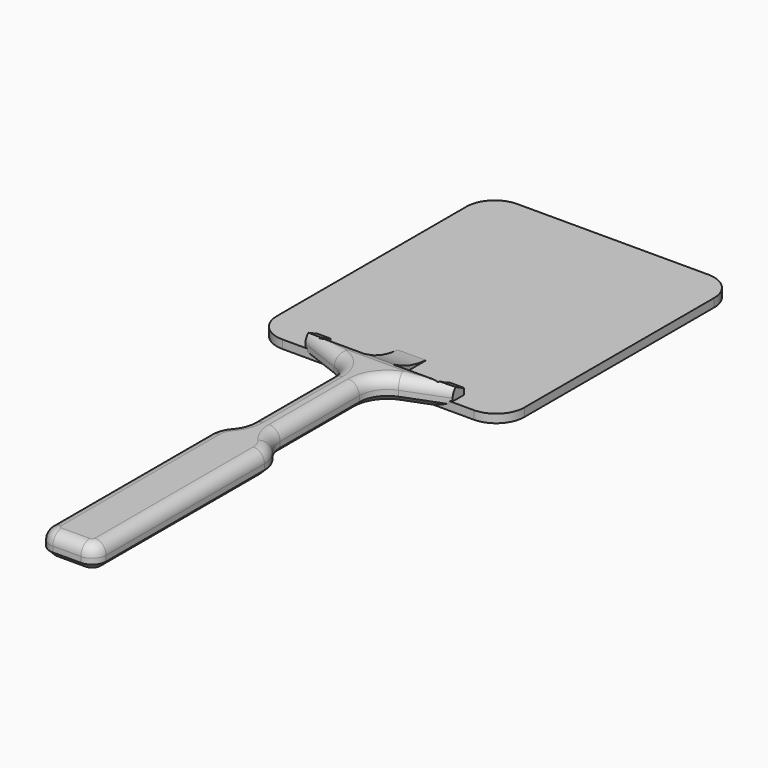
from build123d import *

# Parameters (mm, degrees)
F2_DEPTH      = 3
F1_W          = 10
F1_H          = 50.7820645242
F1_H_2        = 8.1103595249
F1_H_3        = 14.6
F1_W_2        = 5
F1_H_4        = 5
F3_DEPTH      = 8
F4_T1_DEPTH   = 8
F5_R          = 10
F6_R          = 5
F7_R          = 10
F8_R          = 31.9895246327
F9_DEPTH      = 30
F9_DEPTH_BACK = 30
F10_T1_DEPTH  = 44.710583772
F10_T3_DEPTH  = 55.9785297761
F10_T5_DEPTH  = 44.710583772
F10_T7_DEPTH  = 35.23873089
F10_T9_DEPTH  = 70.4314974826
F10_T11_DEPTH = 10
F10_T14_ANGLE = 69.0798918948
F10_T16_ANGLE = 69.0798918948
F10_T18_ANGLE = 41.4096221077
F10_T20_ANGLE = 41.4096221088
F10_T22_ANGLE = 90
F10_T24_ANGLE = 90
F10_T26_ANGLE = 41.4096221088
F10_T28_ANGLE = 41.4096221077
F11_T1_DEPTH  = 70.4314974826
F11_T3_DEPTH  = 35.23873089
F11_T5_DEPTH  = 20.9741913293
F11_T7_DEPTH  = 10
F11_T9_DEPTH  = 20.9741913293
F11_T12_ANGLE = 69.0798918948
F11_T14_ANGLE = 41.4096221077
F11_T16_ANGLE = 41.4096221088
F11_T18_ANGLE = 90
F11_T20_ANGLE = 90
F11_T22_ANGLE = 41.4096221088
F11_T24_ANGLE = 41.4096221077
F11_T26_ANGLE = 69.0798918948


# Not quite as in the source:
# - a fillet or chamfer that OpenCascade refuses, or shapes differently, is made with other operations: its cross-section is extruded or revolved along the edge and cut away or added


with BuildPart() as f2:
    # F0 (on Top) → F2 (new body)
    with BuildSketch(Plane.XY):
        with BuildLine():
            Line((34.0520262078, 104.4403978414), (-34.0520262078, 104.4403978414))
            ThreePointArc((-34.0520262078, 104.4403978414), (-41.1230940197, 101.5114656532), (-44.0520262078, 94.4403978414))
            Line((-44.0520262078, 94.4403978414), (-44.0520262078, 10))
            ThreePointArc((-44.0520262078, 10), (-41.1230940197, 2.9289321881), (-34.0520262078, 0))
            Line((-34.0520262078, 0), (34.0520262078, 0))
            ThreePointArc((34.0520262078, 0), (41.1230940197, 2.9289321881), (44.0520262078, 10))
            Line((44.0520262078, 10), (44.0520262078, 94.4403978414))
            ThreePointArc((44.0520262078, 94.4403978414), (41.1230940197, 101.5114656532), (34.0520262078, 104.4403978414))
        make_face()
    extrude(amount=F2_DEPTH)


with BuildPart() as f3:
    # F1 (on Top) → F3 (new body)
    with BuildSketch(Plane.XY):
        Polygon((5, -58.4924240492), (-5, -58.4924240492), (-10, -58.4924240492), (-10, -138.4924240492), (10, -138.4924240492), (10, -58.4924240492), align=None)
        with Locations((0, -33.1013917871)):
            Rectangle(F1_W, F1_H)
        with Locations((0, -3.6551797625)):
            Rectangle(F1_W, F1_H_2)
        Polygon((-5, -7.7103595249), (-5, 0.4), (-21.2165865879, 0.4), (-26.2165865879, 0.4), align=None)
        Polygon((21.2165865879, 0.4), (5, 0.4), (5, -7.7103595249), (26.2165865879, 0.4), align=None)
        with Locations((0, 7.7)):
            Rectangle(F1_W, F1_H_3)
        with Locations((-23.7165865879, 2.9)):
            Rectangle(F1_W_2, F1_H_4)
        with Locations((23.7165865879, 2.9)):
            Rectangle(F1_W_2, F1_H_4)
    extrude(amount=F3_DEPTH)

    # F4: fillet of radius 10 on 2 edges, made by hand

    # F4_s2 → F4_t1 (join)
    with BuildSketch(Plane.XY):
        with BuildLine():
            ThreePointArc((-10, -58.4924240492), (-6.3397459622, -54.8321700113), (-5, -49.8321700113))
            Line((-5, -49.8321700113), (-5, -58.4924240492))
            Line((-5, -58.4924240492), (-10, -58.4924240492))
        make_face()
        with BuildLine():
            ThreePointArc((10, -58.4924240492), (6.3397459622, -54.8321700113), (5, -49.8321700113))
            Line((5, -49.8321700113), (5, -58.4924240492))
            Line((5, -58.4924240492), (10, -58.4924240492))
        make_face()
    extrude(amount=F4_T1_DEPTH)

    # F5
    f5_edges = [f3.edges().sort_by_distance(p)[0] for p in [
        (10, -58.492424, 4),
        (-10, -58.492424, 4),
    ]]
    fillet(f5_edges, radius=F5_R)

    # F6
    f6_edges = [f3.edges().sort_by_distance(p)[0] for p in [
        (-10, -138.492424, 4),
        (10, -138.492424, 4),
    ]]
    fillet(f6_edges, radius=F6_R)

    # F7
    f7_edges = [f3.edges().sort_by_distance(p)[0] for p in [
        (-5, -7.71036, 4),
        (5, -7.71036, 4),
    ]]
    fillet(f7_edges, radius=F7_R)

    # F8 (on Right) → F9 (cut, two sides)
    with BuildSketch(Plane.YZ) as f9_sk:
        with Locations((17.1725142692, 34.9895246327)):
            Circle(F8_R)
    extrude(amount=-F9_DEPTH, mode=Mode.SUBTRACT)
    extrude(f9_sk.sketch, amount=F9_DEPTH_BACK, mode=Mode.SUBTRACT)

    # F10: fillet of radius 4 on 16 edges, made by hand

    # F10_s2 → F10_t1 (cut)
    with BuildSketch(Plane(origin=(-49.9834696062, 19.1069334895, 0), x_dir=(0, 0, 1), z_dir=(0.9340792186, -0.3570658389, 0))):
        with BuildLine():
            ThreePointArc((4, 8.9874157949), (6.8284271247, 7.8158429197), (8, 4.9874157949))
            Line((8, 4.9874157949), (8, 8.9874157949))
            Line((8, 8.9874157949), (4, 8.9874157949))
        make_face()
    extrude(amount=F10_T1_DEPTH, mode=Mode.SUBTRACT)

    # F10_s4 → F10_t3 (cut)
    with BuildSketch(Plane.YZ.offset(-27.9892648881)):
        with BuildLine():
            ThreePointArc((-1.1276290725, 8), (-0.0733831244, 7.8585703934), (0.9063120288, 7.4442827405))
            ThreePointArc((0.9063120288, 7.4442827405), (0.4508473107, 7.7183761355), (0, 8))
            Line((0, 8), (-1.1276290725, 8))
        make_face()
    extrude(amount=F10_T3_DEPTH, mode=Mode.SUBTRACT)

    # F10_s6 → F10_t5 (cut)
    with BuildSketch(Plane(origin=(8.2202424512, 3.1423113885, 0), x_dir=(0, 0, 1), z_dir=(0.9340792186, 0.3570658389, 0))):
        with BuildLine():
            ThreePointArc((4, 8.9874157949), (6.8284271247, 7.8158429197), (8, 4.9874157949))
            Line((8, 4.9874157949), (8, 8.9874157949))
            Line((8, 8.9874157949), (4, 8.9874157949))
        make_face()
    extrude(amount=F10_T5_DEPTH, mode=Mode.SUBTRACT)

    # F10_s8 → F10_t7 (cut)
    with BuildSketch(Plane.XZ.offset(14.5934391213)):
        with BuildLine():
            ThreePointArc((5, 4), (3.8284271247, 6.8284271247), (1, 8))
            Line((1, 8), (5, 8))
            Line((5, 8), (5, 4))
        make_face()
        with BuildLine():
            ThreePointArc((-5, 4), (-3.8284271247, 6.8284271247), (-1, 8))
            Line((-1, 8), (-5, 8))
            Line((-5, 8), (-5, 4))
        make_face()
    extrude(amount=F10_T7_DEPTH, mode=Mode.SUBTRACT)

    # F10_s10 → F10_t9 (cut)
    with BuildSketch(Plane.XZ.offset(63.0609265666)):
        with BuildLine():
            ThreePointArc((10, 4), (8.8284271247, 6.8284271247), (6, 8))
            Line((6, 8), (10, 8))
            Line((10, 8), (10, 4))
        make_face()
        with BuildLine():
            ThreePointArc((-10, 4), (-8.8284271247, 6.8284271247), (-6, 8))
            Line((-6, 8), (-10, 8))
            Line((-10, 8), (-10, 4))
        make_face()
    extrude(amount=F10_T9_DEPTH, mode=Mode.SUBTRACT)

    # F10_s12 → F10_t11 (cut)
    with BuildSketch(Plane.YZ.offset(-5)):
        with BuildLine():
            ThreePointArc((-138.4924240492, 4), (-137.3208511739, 6.8284271247), (-134.4924240492, 8))
            Line((-134.4924240492, 8), (-138.4924240492, 8))
            Line((-138.4924240492, 8), (-138.4924240492, 4))
        make_face()
    extrude(amount=F10_T11_DEPTH, mode=Mode.SUBTRACT)

    # F10_s13 → F10_t14 (revolve, cut)
    with BuildSketch(Plane.XZ.offset(14.5934391213)):
        with BuildLine():
            ThreePointArc((-5, 4), (-3.8284271247, 6.8284271247), (-1, 8))
            Line((-1, 8), (-5, 8))
            Line((-5, 8), (-5, 4))
        make_face()
    revolve(axis=Axis((-15, -14.5934391213, 8), (0, 0, 1)), revolution_arc=F10_T14_ANGLE, mode=Mode.SUBTRACT)

    # F10_s15 → F10_t16 (revolve, cut)
    with BuildSketch(Plane.XZ.offset(14.5934391213)):
        with BuildLine():
            ThreePointArc((5, 4), (3.8284271247, 6.8284271247), (1, 8))
            Line((1, 8), (5, 8))
            Line((5, 8), (5, 4))
        make_face()
    revolve(axis=Axis((15, -14.5934391213, 8), (0, 0, -1)), revolution_arc=F10_T16_ANGLE, mode=Mode.SUBTRACT)

    # F10_s17 → F10_t18 (revolve, cut)
    with BuildSketch(Plane(origin=(31.2831617138, -35.4717711942, 0), x_dir=(0, 0, 1), z_dir=(0.6614378278, -0.75, 0))):
        with BuildLine():
            ThreePointArc((4, 31.7108822847), (6.8284271247, 32.88245516), (8, 35.7108822847))
            Line((8, 35.7108822847), (8, 31.7108822847))
            Line((8, 31.7108822847), (4, 31.7108822847))
        make_face()
    revolve(axis=Axis((15.0000000004, -49.8321700111, 8), (0, 0, -1)), revolution_arc=F10_T18_ANGLE, mode=Mode.SUBTRACT)

    # F10_s19 → F10_t20 (revolve, cut)
    with BuildSketch(Plane.XZ.offset(63.0609265666)):
        with BuildLine():
            ThreePointArc((10, 4), (8.8284271247, 6.8284271247), (6, 8))
            Line((6, 8), (10, 8))
            Line((10, 8), (10, 4))
        make_face()
    revolve(axis=Axis((0, -63.0609265666, 8), (0, 0, 1)), revolution_arc=F10_T20_ANGLE, mode=Mode.SUBTRACT)

    # F10_s21 → F10_t22 (revolve, cut)
    with BuildSketch(Plane.YZ.offset(5)):
        with BuildLine():
            ThreePointArc((-138.4924240492, 4), (-137.3208511739, 6.8284271247), (-134.4924240492, 8))
            Line((-134.4924240492, 8), (-138.4924240492, 8))
            Line((-138.4924240492, 8), (-138.4924240492, 4))
        make_face()
    revolve(axis=Axis((5, -133.4924240492, 8), (0, 0, 1)), revolution_arc=F10_T22_ANGLE, mode=Mode.SUBTRACT)

    # F10_s23 → F10_t24 (revolve, cut)
    with BuildSketch(Plane.XZ.offset(133.4924240492)):
        with BuildLine():
            ThreePointArc((-10, 4), (-8.8284271247, 6.8284271247), (-6, 8))
            Line((-6, 8), (-10, 8))
            Line((-10, 8), (-10, 4))
        make_face()
    revolve(axis=Axis((-5, -133.4924240492, 8), (0, 0, 1)), revolution_arc=F10_T24_ANGLE, mode=Mode.SUBTRACT)

    # F10_s25 → F10_t26 (revolve, cut)
    with BuildSketch(Plane.XZ.offset(63.0609265666)):
        with BuildLine():
            ThreePointArc((-10, 4), (-8.8284271247, 6.8284271247), (-6, 8))
            Line((-6, 8), (-10, 8))
            Line((-10, 8), (-10, 4))
        make_face()
    revolve(axis=Axis((0, -63.0609265666, 8), (0, 0, -1)), revolution_arc=F10_T26_ANGLE, mode=Mode.SUBTRACT)

    # F10_s27 → F10_t28 (revolve, cut)
    with BuildSketch(Plane(origin=(-31.2831617138, -35.4717711942, 0), x_dir=(0, 0, 1), z_dir=(-0.6614378278, -0.75, 0))):
        with BuildLine():
            ThreePointArc((4, -31.7108822847), (6.8284271247, -32.88245516), (8, -35.7108822847))
            Line((8, -35.7108822847), (8, -31.7108822847))
            Line((8, -31.7108822847), (4, -31.7108822847))
        make_face()
    revolve(axis=Axis((-15.0000000004, -49.8321700111, 8), (0, 0, 1)), revolution_arc=F10_T28_ANGLE, mode=Mode.SUBTRACT)

    # F11: chamfer of 2 on 15 edges, made by hand

    # F11_s2 → F11_t1 (cut)
    with BuildSketch(Plane.XZ.offset(63.0609265666)):
        Polygon((-8, 0), (-10, 2), (-10, 0), align=None)
        Polygon((8, 0), (10, 2), (10, 0), align=None)
    extrude(amount=F11_T1_DEPTH, mode=Mode.SUBTRACT)

    # F11_s4 → F11_t3 (cut)
    with BuildSketch(Plane.XZ.offset(14.5934391213)):
        Polygon((-3, 0), (-5, 2), (-5, 0), align=None)
        Polygon((3, 0), (5, 2), (5, 0), align=None)
    extrude(amount=F11_T3_DEPTH, mode=Mode.SUBTRACT)

    # F11_s6 → F11_t5 (cut)
    with BuildSketch(Plane(origin=(-27.8117986999, 10.6314786102, 0), x_dir=(0, 0, 1), z_dir=(0.9340792186, -0.3570658389, 0))):
        Polygon((0, 6.9874157949), (2, 8.9874157949), (0, 8.9874157949), align=None)
    extrude(amount=F11_T5_DEPTH, mode=Mode.SUBTRACT)

    # F11_s8 → F11_t7 (cut)
    with BuildSketch(Plane.YZ.offset(-5)):
        Polygon((-136.4924240492, 0), (-138.4924240492, 2), (-138.4924240492, 0), align=None)
    extrude(amount=F11_T7_DEPTH, mode=Mode.SUBTRACT)

    # F11_s10 → F11_t9 (cut)
    with BuildSketch(Plane(origin=(8.2202424512, 3.1423113885, 0), x_dir=(0, 0, 1), z_dir=(0.9340792186, 0.3570658389, 0))):
        Polygon((0, 6.9874157949), (2, 8.9874157949), (0, 8.9874157949), align=None)
    extrude(amount=F11_T9_DEPTH, mode=Mode.SUBTRACT)

    # F11_s11 → F11_t12 (revolve, cut)
    with BuildSketch(Plane.XZ.offset(14.5934391213)):
        Polygon((-3, 0), (-5, 2), (-5, 0), align=None)
    revolve(axis=Axis((-15, -14.5934391213, 0), (0, 0, 1)), revolution_arc=F11_T12_ANGLE, mode=Mode.SUBTRACT)

    # F11_s13 → F11_t14 (revolve, cut)
    with BuildSketch(Plane(origin=(-31.2831617138, -35.4717711942, 0), x_dir=(0, 0, 1), z_dir=(-0.6614378278, -0.75, 0))):
        Polygon((0, -33.7108822847), (2, -31.7108822847), (0, -31.7108822847), align=None)
    revolve(axis=Axis((-15.0000000004, -49.8321700111, 0), (0, 0, 1)), revolution_arc=F11_T14_ANGLE, mode=Mode.SUBTRACT)

    # F11_s15 → F11_t16 (revolve, cut)
    with BuildSketch(Plane.XZ.offset(63.0609265666)):
        Polygon((-8, 0), (-10, 2), (-10, 0), align=None)
    revolve(axis=Axis((0, -63.0609265666, 0), (0, 0, -1)), revolution_arc=F11_T16_ANGLE, mode=Mode.SUBTRACT)

    # F11_s17 → F11_t18 (revolve, cut)
    with BuildSketch(Plane.XZ.offset(133.4924240492)):
        Polygon((-8, 0), (-10, 2), (-10, 0), align=None)
    revolve(axis=Axis((-5, -133.4924240492, 0), (0, 0, 1)), revolution_arc=F11_T18_ANGLE, mode=Mode.SUBTRACT)

    # F11_s19 → F11_t20 (revolve, cut)
    with BuildSketch(Plane.YZ.offset(5)):
        Polygon((-136.4924240492, 0), (-138.4924240492, 2), (-138.4924240492, 0), align=None)
    revolve(axis=Axis((5, -133.4924240492, 0), (0, 0, 1)), revolution_arc=F11_T20_ANGLE, mode=Mode.SUBTRACT)

    # F11_s21 → F11_t22 (revolve, cut)
    with BuildSketch(Plane.XZ.offset(63.0609265666)):
        Polygon((8, 0), (10, 2), (10, 0), align=None)
    revolve(axis=Axis((0, -63.0609265666, 0), (0, 0, 1)), revolution_arc=F11_T22_ANGLE, mode=Mode.SUBTRACT)

    # F11_s23 → F11_t24 (revolve, cut)
    with BuildSketch(Plane(origin=(31.2831617138, -35.4717711942, 0), x_dir=(0, 0, 1), z_dir=(0.6614378278, -0.75, 0))):
        Polygon((0, 33.7108822847), (2, 31.7108822847), (0, 31.7108822847), align=None)
    revolve(axis=Axis((15.0000000004, -49.8321700111, 0), (0, 0, -1)), revolution_arc=F11_T24_ANGLE, mode=Mode.SUBTRACT)

    # F11_s25 → F11_t26 (revolve, cut)
    with BuildSketch(Plane.XZ.offset(14.5934391213)):
        Polygon((3, 0), (5, 2), (5, 0), align=None)
    revolve(axis=Axis((15, -14.5934391213, 0), (0, 0, -1)), revolution_arc=F11_T26_ANGLE, mode=Mode.SUBTRACT)


solid = Compound([f2.part, f3.part])
